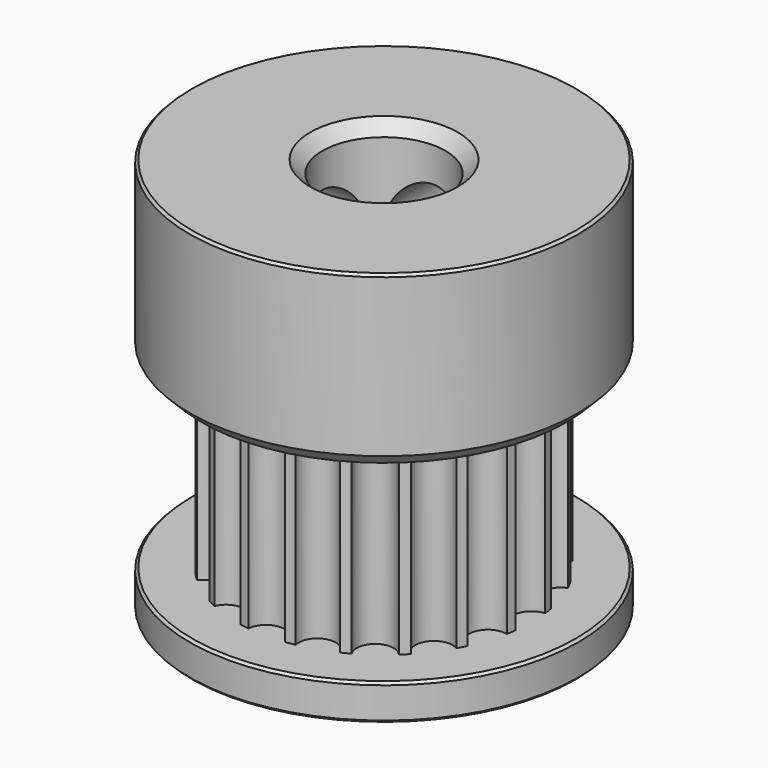
from build123d import *

# Parameters (mm, degrees)
F0_R            = 7.9
F1_DEPTH        = 1.46
F2_R            = 6
F3_DEPTH        = 7.6
F4_R            = 0.75
F5_DEPTH        = 7.6
F5_COPIES_COUNT = 20
F6_R            = 7.9
F7_DEPTH        = 7
F8_R            = 1.5
F9_DEPTH        = 25
F9_COPIES_COUNT = 2
F9_COPIES_ANGLE = 90
F10_R           = 2.5
F11_DEPTH       = 25
F12_SIZE        = 0.5
F13_SIZE        = 0.1


# Not quite as in the source:
# - a pattern or mirror of a feature is missing from the dataset's text; its kind, count and spacing are read off the source's solid


with BuildPart() as f1:
    # F0 (on Top) → F1 (new body)
    with BuildSketch(Plane.XY):
        Circle(F0_R)
    extrude(amount=F1_DEPTH)

    # F2 (on face) → F3 (join)
    with BuildSketch(Plane.XY.offset(1.46)):
        Circle(F2_R)
    extrude(amount=F3_DEPTH)

    # F4 (on face) → F5 (cut)
    with BuildSketch(Plane.XY.offset(9.06)):
        with Locations((0, -6)):
            Circle(F4_R)
    f5 = extrude(amount=-F5_DEPTH, mode=Mode.SUBTRACT)

    # F5_copies: F5 ×20 about axis
    f5_copies_axis = Axis((0, 0, 0), (0, 0, 1))
    for i in range(1, F5_COPIES_COUNT):
        add(f5.rotate(f5_copies_axis, i * 360 / F5_COPIES_COUNT), mode=Mode.SUBTRACT)

    # F6 (on face) → F7 (join)
    with BuildSketch(Plane.XY.offset(9.06)):
        Circle(F6_R)
    extrude(amount=F7_DEPTH)

    # F8 (on Front) → F9 (cut)
    with BuildSketch(Plane.XZ):
        with Locations((0, 12.66)):
            Circle(F8_R)
    f9 = extrude(amount=-F9_DEPTH, mode=Mode.SUBTRACT)

    # F9_copies: F9 ×2 about axis
    f9_copies_axis = Axis((0, 0, 0), (0, 0, 1))
    for i in range(1, F9_COPIES_COUNT):
        add(f9.rotate(f9_copies_axis, i * F9_COPIES_ANGLE / (F9_COPIES_COUNT - 1)), mode=Mode.SUBTRACT)

    # F10 (on face) → F11 (cut)
    with BuildSketch(Plane.XY.offset(16.06)):
        Circle(F10_R)
    extrude(amount=-F11_DEPTH, mode=Mode.SUBTRACT)

    # F12
    f12_edges = [f1.edges().sort_by_distance(p)[0] for p in [
        (-7.9, 0, 9.06),
        (-2.5, 0, 0),
        (-2.5, 0, 16.06),
    ]]
    chamfer(f12_edges, length=F12_SIZE)

    # F13
    f13_edges = [f1.edges().sort_by_distance(p)[0] for p in [
        (-7.9, 0, 0),
        (-7.9, 0, 1.46),
        (-7.9, 0, 16.06),
    ]]
    chamfer(f13_edges, length=F13_SIZE)


solid = f1.part
